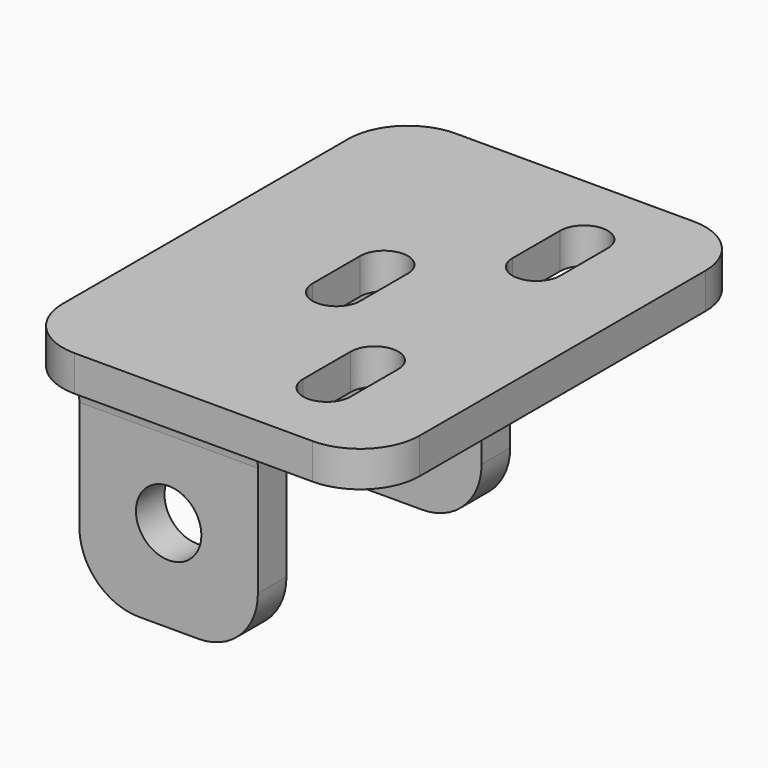
from build123d import *

# Parameters (mm, degrees)
F2_W        = 15
F2_H        = 19.25
F2_R        = 2.75
F3_DEPTH    = 40
F5_DEPTH    = 22.251
F6_W        = 6.75
F6_H        = 19.25
F6_W_2      = 20.5
F7_DEPTH    = 30.001
F8_T1_DEPTH = 15
F8_T3_DEPTH = 28
F8_T5_DEPTH = 28
F8_T7_DEPTH = 28
F10_R       = 2


# Not quite as in the source:
# - a fillet or chamfer that OpenCascade refuses, or shapes differently, is made with other operations: its cross-section is extruded or revolved along the edge and cut away or added
# - a feature of the source that left no trace in its solid (it failed there, or was rolled back) is left out


with BuildPart() as f3:
    # F2 (on Front) → F3 (new body)
    with BuildSketch(Plane.XZ):
        Polygon((-47, -12.4571), (-32, -12.4571), (-17, -12.4571), (-17, -9.4571), (-47, -9.4571), align=None)
        with Locations((-39.5, -22.0821)):
            Rectangle(F2_W, F2_H)
        with Locations((-39.5, -23.9571)):
            Circle(F2_R, mode=Mode.SUBTRACT)
    extrude(amount=F3_DEPTH)

    # F4 (on face) → F5 (cut, through all)
    with BuildSketch(Plane.XY.offset(-9.4571)):
        with BuildLine():
            Line((-24, -11.5), (-24, -6.5))
            ThreePointArc((-24, -6.5), (-26, -4.5), (-28, -6.5))
            Line((-28, -6.5), (-28, -11.5))
            ThreePointArc((-28, -11.5), (-26, -13.5), (-24, -11.5))
        make_face()
        with BuildLine():
            Line((-32, -22.5), (-32, -17.5))
            ThreePointArc((-32, -17.5), (-34, -15.5), (-36, -17.5))
            Line((-36, -17.5), (-36, -22.5))
            ThreePointArc((-36, -22.5), (-34, -24.5), (-32, -22.5))
        make_face()
        with BuildLine():
            ThreePointArc((-28, -33.5), (-26, -35.5), (-24, -33.5))
            Line((-24, -33.5), (-24, -28.5))
            ThreePointArc((-24, -28.5), (-26, -26.5), (-28, -28.5))
            Line((-28, -28.5), (-28, -33.5))
        make_face()
    extrude(amount=-F5_DEPTH, mode=Mode.SUBTRACT)

    # F6 (on face) → F7 (cut, through all)
    with BuildSketch(Plane(origin=(-47, 0, 0), x_dir=(0, -1, 0), z_dir=(-1, 0, 0))):
        with Locations((3.375, -22.0821)):
            Rectangle(F6_W, F6_H)
        with Locations((20, -22.0821)):
            Rectangle(F6_W_2, F6_H)
        with Locations((36.625, -22.0821)):
            Rectangle(F6_W, F6_H)
    extrude(amount=-F7_DEPTH, mode=Mode.SUBTRACT)

    # F8: fillet of radius 5 on 10 edges, made by hand

    # F8_s2 → F8_t1 (join)
    with BuildSketch(Plane.YZ.offset(-47)):
        with BuildLine():
            ThreePointArc((-1.75, -12.4571), (-5.2855339059, -13.9215660941), (-6.75, -17.4571))
            Line((-6.75, -17.4571), (-6.75, -12.4571))
            Line((-6.75, -12.4571), (-1.75, -12.4571))
        make_face()
        with BuildLine():
            ThreePointArc((-38.25, -12.4571), (-34.7144660941, -13.9215660941), (-33.25, -17.4571))
            Line((-33.25, -17.4571), (-33.25, -12.4571))
            Line((-33.25, -12.4571), (-38.25, -12.4571))
        make_face()
    extrude(amount=F8_T1_DEPTH)

    # F8_s4 → F8_t3 (cut)
    with BuildSketch(Plane.XY.offset(-24.9571)):
        with BuildLine():
            ThreePointArc((-17, -5), (-18.4644660941, -1.4644660941), (-22, 0))
            Line((-22, 0), (-17, 0))
            Line((-17, 0), (-17, -5))
        make_face()
        with BuildLine():
            ThreePointArc((-17, -35), (-18.4644660941, -38.5355339059), (-22, -40))
            Line((-22, -40), (-17, -40))
            Line((-17, -40), (-17, -35))
        make_face()
        with BuildLine():
            ThreePointArc((-47, -5), (-45.5355339059, -1.4644660941), (-42, 0))
            Line((-42, 0), (-47, 0))
            Line((-47, 0), (-47, -5))
        make_face()
        with BuildLine():
            ThreePointArc((-42, -40), (-45.5355339059, -38.5355339059), (-47, -35))
            Line((-47, -35), (-47, -40))
            Line((-47, -40), (-42, -40))
        make_face()
    extrude(amount=F8_T3_DEPTH, mode=Mode.SUBTRACT)

    # F8_s6 → F8_t5 (cut)
    with BuildSketch(Plane.XZ.offset(17.75)):
        with BuildLine():
            ThreePointArc((-42, -31.7071), (-45.5355339059, -30.2426339059), (-47, -26.7071))
            Line((-47, -26.7071), (-47, -31.7071))
            Line((-47, -31.7071), (-42, -31.7071))
        make_face()
        with BuildLine():
            ThreePointArc((-37, -31.7071), (-33.4644660941, -30.2426339059), (-32, -26.7071))
            Line((-32, -26.7071), (-32, -31.7071))
            Line((-32, -31.7071), (-37, -31.7071))
        make_face()
    extrude(amount=F8_T5_DEPTH, mode=Mode.SUBTRACT)

    # F8_s8 → F8_t7 (cut)
    with BuildSketch(Plane.XZ.offset(-5.75)):
        with BuildLine():
            ThreePointArc((-42, -31.7071), (-45.5355339059, -30.2426339059), (-47, -26.7071))
            Line((-47, -26.7071), (-47, -31.7071))
            Line((-47, -31.7071), (-42, -31.7071))
        make_face()
        with BuildLine():
            ThreePointArc((-37, -31.7071), (-33.4644660941, -30.2426339059), (-32, -26.7071))
            Line((-32, -26.7071), (-32, -31.7071))
            Line((-32, -31.7071), (-37, -31.7071))
        make_face()
    extrude(amount=F8_T7_DEPTH, mode=Mode.SUBTRACT)

    # F10
    f10_edges = [f3.edges().sort_by_distance(p)[0] for p in [
        (-39.5, -30.25, -12.4571),
        (-39.5, -9.75, -12.4571),
        (-32, -34.25, -12.4571),
        (-32, -5.75, -12.4571),
    ]]
    fillet(f10_edges, radius=F10_R)


solid = f3.part
